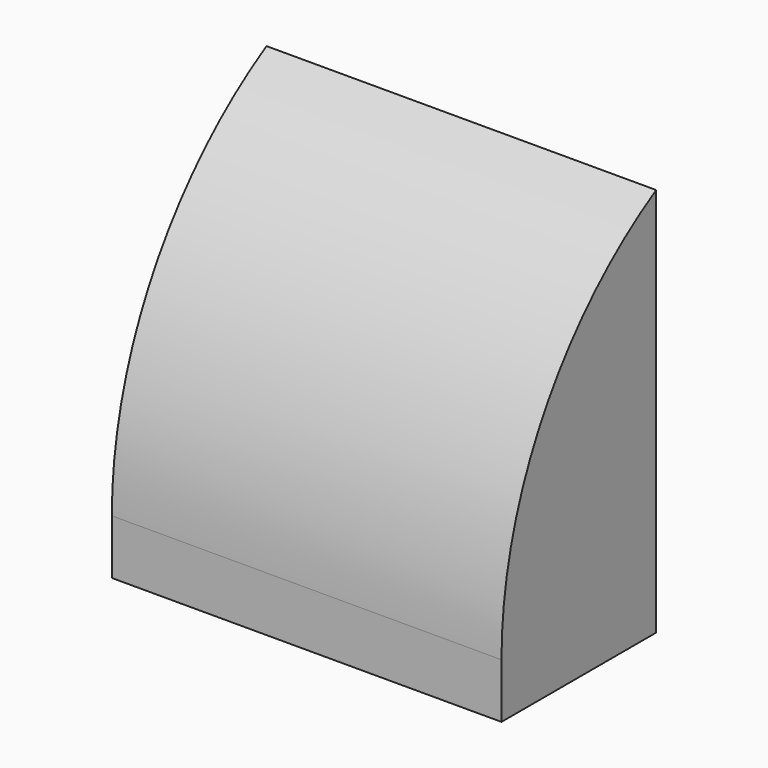
from build123d import *

# Parameters (mm, degrees)
F0_W        = 51.1865206063
F0_H        = 51.1865206063
F1_DEPTH    = 25.4
F2_T1_DEPTH = 271.1569731675


# Not quite as in the source:
# - a fillet or chamfer that OpenCascade refuses, or shapes differently, is made with other operations: its cross-section is extruded or revolved along the edge and cut away or added


with BuildPart() as f1:
    # F0 (on Front) → F1 (new body)
    with BuildSketch(Plane.XZ):
        with Locations((-25.5932603031, 30.0658736378)):
            Rectangle(F0_W, F0_H)
    extrude(amount=F1_DEPTH)

    # F2: fillet of radius 50.8 on 1 edges, made by hand

    # F2_s2 → F2_t1 (cut)
    with BuildSketch(Plane.YZ.offset(-161.1717468869)):
        with BuildLine():
            ThreePointArc((0, 55.6591339409), (-18.5940905122, 37.0650434287), (-25.4, 11.6650434287))
            Line((-25.4, 11.6650434287), (-25.4, 55.6591339409))
            Line((-25.4, 55.6591339409), (0, 55.6591339409))
        make_face()
    extrude(amount=F2_T1_DEPTH, mode=Mode.SUBTRACT)


solid = f1.part
